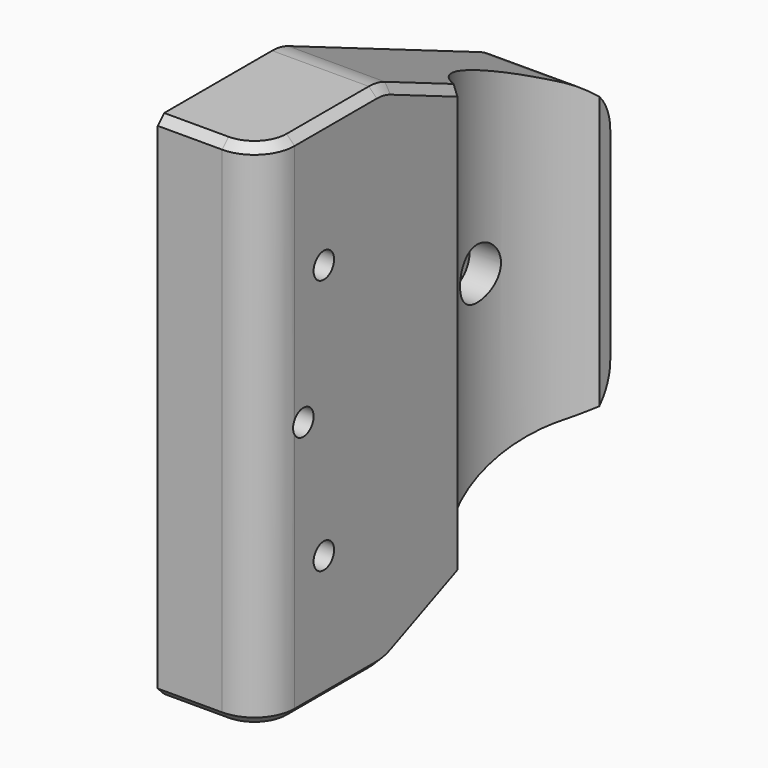
from build123d import *

# Parameters (mm, degrees)
F0_R        = 1.5875
F0_R_2      = 3.175
F1_DEPTH    = 13
F3_DEPTH    = 37.5
F4_R        = 6.35
F5_T1_DEPTH = 88.5
F6_SIZE     = 1
F7_SIZE     = 3.175


# Not quite as in the source:
# - a fillet or chamfer that OpenCascade refuses, or shapes differently, is made with other operations: its cross-section is extruded or revolved along the edge and cut away or added
# - a feature names something its author has since deleted; it is built from what else it names


with BuildPart() as f1:
    # F0 (on Right) → F1 (new body)
    with BuildSketch(Plane.YZ):
        Polygon((0, 31.75), (0, 0), (0, -31.75), (19.05, -31.75), (53.975, -16.7821428571), (53.975, 16.7821428571), (19.05, 31.75), align=None)
        with Locations((9.525, -15.875)):
            Circle(F0_R, mode=Mode.SUBTRACT)
        with Locations((6.35, 0)):
            Circle(F0_R, mode=Mode.SUBTRACT)
        with Locations((9.525, 15.875)):
            Circle(F0_R, mode=Mode.SUBTRACT)
        with Locations((41.275, 0)):
            Circle(F0_R_2, mode=Mode.SUBTRACT)
    extrude(amount=-F1_DEPTH)

    # F2 (on Top) → F3 (cut, symmetric)
    with BuildSketch(Plane.XY):
        with BuildLine():
            Line((0, 30.2764773719), (0, 52.2735226281))
            ThreePointArc((0, 52.2735226281), (-6.35, 41.275), (0, 30.2764773719))
        make_face()
    extrude(amount=F3_DEPTH, both=True, mode=Mode.SUBTRACT)

    # F4
    f4_edges = [f1.edges().sort_by_distance(p)[0] for p in [
        (-6.5, 19.05, 31.75),
        (-6.5, 19.05, -31.75),
        (-6.5, 53.975, 16.782143),
        (-6.5, 53.975, -16.782143),
    ]]
    fillet(f4_edges, radius=F4_R)

    # F5: fillet of radius 5 on 1 edges, made by hand

    # F5_s2 → F5_t1 (cut)
    with BuildSketch(Plane.XY.offset(-44.25)):
        with BuildLine():
            ThreePointArc((0, 5), (-1.4644660941, 1.4644660941), (-5, 0))
            Line((-5, 0), (0, 0))
            Line((0, 0), (0, 5))
        make_face()
    extrude(amount=F5_T1_DEPTH, mode=Mode.SUBTRACT)

    # F6
    f6_edges = [f1.edges().sort_by_distance(p)[0] for p in [
        (0, 11.373307, 31.75),
        (0, 25.262239, -29.087612),
        (0, 25.262239, 29.087612),
        (0, 19.023382, -31.620319),
        (0, 11.373307, -31.75),
        (0, 19.023382, 31.620319),
        (-9, 0, -31.75),
        (-1.464466, 1.464466, -31.75),
        (-1.464466, 1.464466, 31.75),
        (-9, 0, 31.75),
    ]]
    chamfer(f6_edges, length=F6_SIZE)

    # F7
    f7_edges = [f1.edges().sort_by_distance(p)[0] for p in [
        (-13, 38.1, 0),
    ]]
    chamfer(f7_edges, length=F7_SIZE)


solid = f1.part
